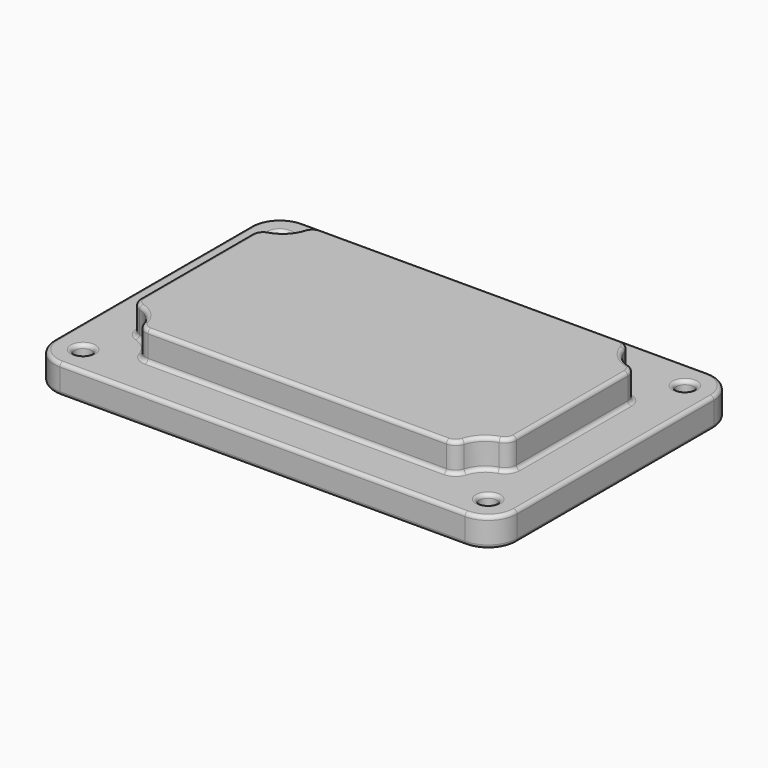
from build123d import *

# Parameters (mm, degrees)
F1_DEPTH  = 6.35
F3_DEPTH  = 6.35
F4_R      = 1.905
F5_DEPTH  = 12.701
F6_R      = 0.8128
F8_DEPTH  = 3.175
F10_DEPTH = 6.35


with BuildPart() as f1:
    # F0 (on Top) → F1 (new body)
    with BuildSketch(Plane.XY):
        with BuildLine():
            ThreePointArc((50.8, 26.9875), (48.9401280605, 31.4776280605), (44.45, 33.3375))
            Line((44.45, 33.3375), (-44.45, 33.3375))
            ThreePointArc((-44.45, 33.3375), (-48.9401280605, 31.4776280605), (-50.8, 26.9875))
            Line((-50.8, 26.9875), (-50.8, -26.9875))
            ThreePointArc((-50.8, -26.9875), (-48.9401280605, -31.4776280605), (-44.45, -33.3375))
            Line((-44.45, -33.3375), (44.45, -33.3375))
            ThreePointArc((44.45, -33.3375), (48.9401280605, -31.4776280605), (50.8, -26.9875))
            Line((50.8, -26.9875), (50.8, 26.9875))
        make_face()
    extrude(amount=F1_DEPTH)

    # F2 (on face) → F3 (join)
    with BuildSketch(Plane.XY.offset(6.35)):
        with BuildLine():
            ThreePointArc((35.1897007184, 21.9982142857), (34.2735213396, 23.3090306634), (32.7555810057, 23.8125))
            Line((32.7555810057, 23.8125), (-32.7555810057, 23.8125))
            ThreePointArc((-32.7555810057, 23.8125), (-34.2735213396, 23.3090306634), (-35.1897007184, 21.9982142857))
            ThreePointArc((-35.1897007184, 21.9982142857), (-36.7848719395, 19.3223719395), (-39.4607142857, 17.7272007184))
            ThreePointArc((-39.4607142857, 17.7272007184), (-40.7715306634, 16.8110213396), (-41.275, 15.2930810057))
            Line((-41.275, 15.2930810057), (-41.275, -15.2930810057))
            ThreePointArc((-41.275, -15.2930810057), (-40.7715306634, -16.8110213396), (-39.4607142857, -17.7272007184))
            ThreePointArc((-39.4607142857, -17.7272007184), (-36.7848719395, -19.3223719395), (-35.1897007184, -21.9982142857))
            ThreePointArc((-35.1897007184, -21.9982142857), (-34.2735213396, -23.3090306634), (-32.7555810057, -23.8125))
            Line((-32.7555810057, -23.8125), (32.7555810057, -23.8125))
            ThreePointArc((32.7555810057, -23.8125), (34.2735213396, -23.3090306634), (35.1897007184, -21.9982142857))
            ThreePointArc((35.1897007184, -21.9982142857), (36.7848719395, -19.3223719395), (39.4607142857, -17.7272007184))
            ThreePointArc((39.4607142857, -17.7272007184), (40.7715306634, -16.8110213396), (41.275, -15.2930810057))
            Line((41.275, -15.2930810057), (41.275, 15.2930810057))
            ThreePointArc((41.275, 15.2930810057), (40.7715306634, 16.8110213396), (39.4607142857, 17.7272007184))
            ThreePointArc((39.4607142857, 17.7272007184), (36.7848719395, 19.3223719395), (35.1897007184, 21.9982142857))
        make_face()
    extrude(amount=F3_DEPTH)

    # F4 (on Top) → F5 (cut, through all)
    with BuildSketch(Plane.XY):
        with Locations((-44.45, 26.9875)):
            Circle(F4_R)
        with Locations((44.45, 26.9875)):
            Circle(F4_R)
        with Locations((44.45, -26.9875)):
            Circle(F4_R)
        with Locations((-44.45, -26.9875)):
            Circle(F4_R)
    extrude(amount=F5_DEPTH, mode=Mode.SUBTRACT)

    # F6
    f6_edges = [f1.edges().sort_by_distance(p)[0] for p in [
        (48.940128, 31.477628, 6.35),
        (50.8, 0, 6.35),
        (0, 33.3375, 6.35),
        (48.940128, -31.477628, 6.35),
        (-48.940128, 31.477628, 6.35),
        (0, -33.3375, 6.35),
        (-50.8, 0, 6.35),
        (-48.940128, -31.477628, 6.35),
        (-46.355, -26.9875, 6.35),
        (42.545, -26.9875, 6.35),
        (36.784872, 19.322372, 6.35),
        (40.771531, 16.811021, 6.35),
        (34.273521, 23.309031, 6.35),
        (41.275, 0, 6.35),
        (0, 23.8125, 6.35),
        (40.771531, -16.811021, 6.35),
        (-34.273521, 23.309031, 6.35),
        (36.784872, -19.322372, 6.35),
        (-36.784872, 19.322372, 6.35),
        (34.273521, -23.309031, 6.35),
        (-40.771531, 16.811021, 6.35),
        (0, -23.8125, 6.35),
        (-41.275, 0, 6.35),
        (-34.273521, -23.309031, 6.35),
        (-40.771531, -16.811021, 6.35),
        (-36.784872, -19.322372, 6.35),
        (-46.355, 26.9875, 6.35),
        (42.545, 26.9875, 6.35),
        (32.755581, -23.8125, 9.525),
        (35.189701, -21.998214, 9.525),
        (34.273521, -23.309031, 12.7),
        (41.275, 15.293081, 9.525),
        (39.460714, 17.727201, 9.525),
        (40.771531, 16.811021, 12.7),
        (39.460714, -17.727201, 9.525),
        (41.275, -15.293081, 9.525),
        (40.771531, -16.811021, 12.7),
        (32.755581, 23.8125, 9.525),
        (-32.755581, 23.8125, 9.525),
        (0, 23.8125, 12.7),
        (36.784872, 19.322372, 12.7),
        (34.273521, 23.309031, 12.7),
        (-34.273521, 23.309031, 12.7),
        (-36.784872, 19.322372, 12.7),
        (-40.771531, 16.811021, 12.7),
        (-41.275, 0, 12.7),
        (-40.771531, -16.811021, 12.7),
        (-36.784872, -19.322372, 12.7),
        (-34.273521, -23.309031, 12.7),
        (0, -23.8125, 12.7),
        (36.784872, -19.322372, 12.7),
        (41.275, 0, 12.7),
        (-32.755581, -23.8125, 9.525),
        (-41.275, 15.293081, 9.525),
        (-41.275, -15.293081, 9.525),
        (-39.460714, -17.727201, 9.525),
        (-35.189701, -21.998214, 9.525),
        (-39.460714, 17.727201, 9.525),
        (-35.189701, 21.998214, 9.525),
        (35.189701, 21.998214, 9.525),
        (44.45, 33.3375, 3.175),
        (-44.45, 33.3375, 3.175),
        (0, 33.3375, 0),
        (-44.45, -33.3375, 3.175),
        (44.45, -33.3375, 3.175),
        (0, -33.3375, 0),
        (50.8, -26.9875, 3.175),
        (50.8, 26.9875, 3.175),
        (50.8, 0, 0),
        (-50.8, 26.9875, 3.175),
        (-50.8, -26.9875, 3.175),
        (-50.8, 0, 0),
        (-48.940128, 31.477628, 0),
        (48.940128, 31.477628, 0),
        (48.940128, -31.477628, 0),
        (-48.940128, -31.477628, 0),
        (-46.355, -26.9875, 0),
        (42.545, -26.9875, 0),
        (-46.355, 26.9875, 0),
        (42.545, 26.9875, 0),
        (46.355, 26.9875, 3.175),
        (-42.545, -26.9875, 3.175),
        (46.355, -26.9875, 3.175),
        (-42.545, 26.9875, 3.175),
    ]]
    fillet(f6_edges, radius=F6_R)

    # F7 (on Top) → F8 (cut)
    with BuildSketch(Plane.XY):
        with BuildLine():
            Line((-40.8022027194, -30.1625), (40.8022027194, -30.1625))
            ThreePointArc((40.8022027194, -30.1625), (41.3650700598, -29.8214478817), (41.3233166167, -29.1646428571))
            ThreePointArc((41.3233166167, -29.1646428571), (41.7559231637, -24.2934231637), (46.6271428571, -23.8608166167))
            ThreePointArc((46.6271428571, -23.8608166167), (47.2839478817, -23.9025700598), (47.625, -23.3397027194))
            Line((47.625, -23.3397027194), (47.625, 23.3397027194))
            ThreePointArc((47.625, 23.3397027194), (47.2839478817, 23.9025700598), (46.6271428571, 23.8608166167))
            ThreePointArc((46.6271428571, 23.8608166167), (41.7559231637, 24.2934231637), (41.3233166167, 29.1646428571))
            ThreePointArc((41.3233166167, 29.1646428571), (41.3650700598, 29.8214478817), (40.8022027194, 30.1625))
            Line((40.8022027194, 30.1625), (-40.8022027194, 30.1625))
            ThreePointArc((-40.8022027194, 30.1625), (-41.3650700598, 29.8214478817), (-41.3233166167, 29.1646428571))
            ThreePointArc((-41.3233166167, 29.1646428571), (-41.7559231637, 24.2934231637), (-46.6271428571, 23.8608166167))
            ThreePointArc((-46.6271428571, 23.8608166167), (-47.2839478817, 23.9025700598), (-47.625, 23.3397027194))
            Line((-47.625, 23.3397027194), (-47.625, -23.3397027194))
            ThreePointArc((-47.625, -23.3397027194), (-47.2839478817, -23.9025700598), (-46.6271428571, -23.8608166167))
            ThreePointArc((-46.6271428571, -23.8608166167), (-41.7559231637, -24.2934231637), (-41.3233166167, -29.1646428571))
            ThreePointArc((-41.3233166167, -29.1646428571), (-41.3650700598, -29.8214478817), (-40.8022027194, -30.1625))
        make_face()
    extrude(amount=F8_DEPTH, mode=Mode.SUBTRACT)

    # F9 (on face) → F10 (cut, through all)
    with BuildSketch(Plane(origin=(0, 0, 3.175), x_dir=(1, 0, 0), z_dir=(0, 0, -1))):
        with BuildLine():
            Line((38.1, -14.8322438789), (38.1, 14.8322438789))
            ThreePointArc((38.1, 14.8322438789), (34.5398079092, 17.0773079092), (32.2947438789, 20.6375))
            Line((32.2947438789, 20.6375), (-32.2947438789, 20.6375))
            ThreePointArc((-32.2947438789, 20.6375), (-34.5398079092, 17.0773079092), (-38.1, 14.8322438789))
            Line((-38.1, 14.8322438789), (-38.1, -14.8322438789))
            ThreePointArc((-38.1, -14.8322438789), (-34.5398079092, -17.0773079092), (-32.2947438789, -20.6375))
            Line((-32.2947438789, -20.6375), (32.2947438789, -20.6375))
            ThreePointArc((32.2947438789, -20.6375), (34.5398079092, -17.0773079092), (38.1, -14.8322438789))
        make_face()
    extrude(amount=-F10_DEPTH, mode=Mode.SUBTRACT)


solid = f1.part
